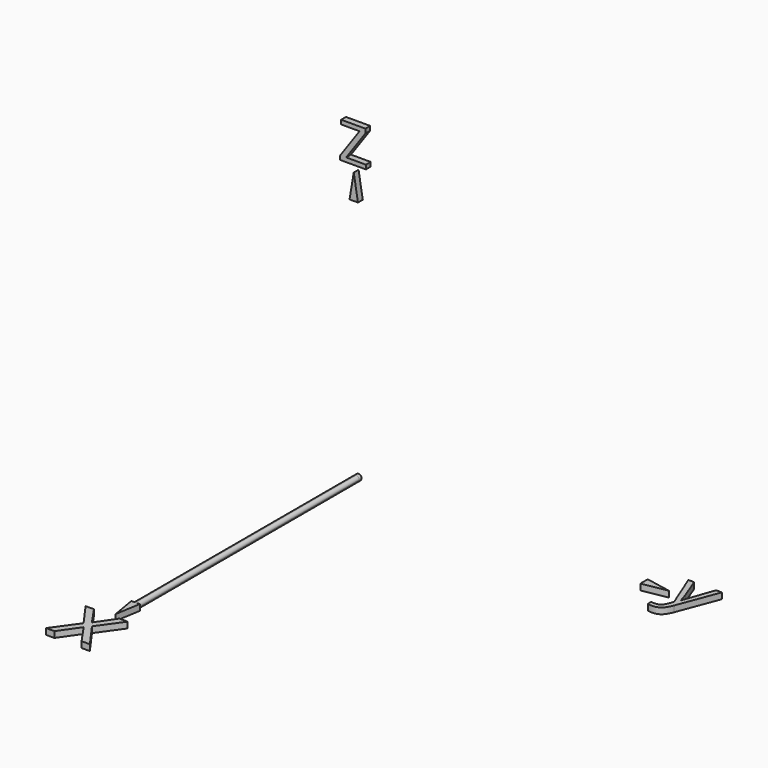
from build123d import *

# Parameters (mm, degrees)
F1_TEXT_SIZE   = 11.1111111111
F3_DEPTH       = 0.5
F0_TEXT_SIZE   = 15.0063579108
F4_DEPTH       = 1
F0_TEXT_SIZE_2 = 11.1111111111
F5_DEPTH       = 1
F6_DEPTH       = 47
F10_DEPTH      = 0.5
F11_DEPTH      = 0.5


# Not quite as in the source:
# - the program builds the solid bodies; features that only make, move or delete a surface that nothing else refers to are left out
# - Text() gives the source's letters only with a copy of the font that has no kerning and outlines rounded to 1/6400 em; it was checked with that copy


with BuildPart() as f3:
    # F1 (on Front) → F3 (new body, symmetric)
    with BuildSketch(Plane.XZ):
        Polygon((-0.699351976, 40.8282129952), (0, 40.8282129952), (0, 45), align=None)
        Polygon((0, 45), (0, 40.8282129952), (0.699351976, 40.8282129952), align=None)
        with BuildLine():
            ThreePointArc((0.5, 0), (0.3535533906, 0.3535533906), (0, 0.5))
            ThreePointArc((0, 0.5), (-0.3535533906, -0.3535533906), (0.5, 0))
        make_face()
        with Locations((-2.7395833333, 46.0987785351)):
            Text('z', F1_TEXT_SIZE, font='Open Sans', text_align=(TextAlign.LEFT, TextAlign.BOTTOM))
    extrude(amount=F3_DEPTH, both=True)


with BuildPart() as f4:
    # F0 (on Top) → F4 (new body)
    with BuildSketch(Plane.XY):
        with Locations((-4.2674330309, -59.449518038)):
            Text('x', F0_TEXT_SIZE, font='Open Sans', text_align=(TextAlign.LEFT, TextAlign.BOTTOM))
    extrude(amount=F4_DEPTH)


with BuildPart() as f5:
    # F0 (on Top) → F5 (new body)
    with BuildSketch(Plane.XY):
        with Locations((52.6564974968, -2.7562453453)):
            Text('y', F0_TEXT_SIZE_2, font='Open Sans', text_align=(TextAlign.LEFT, TextAlign.BOTTOM))
    extrude(amount=F5_DEPTH)


with BuildPart() as f6:
    # F1 (on Front) → F6 (new body)
    with BuildSketch(Plane.XZ):
        with BuildLine():
            ThreePointArc((0.5, 0), (0.3535533906, 0.3535533906), (0, 0.5))
            ThreePointArc((0, 0.5), (-0.3535533906, -0.3535533906), (0.5, 0))
        make_face()
    extrude(amount=F6_DEPTH)

    # F0 (on Top) → F10 (join, symmetric)
    with BuildSketch(Plane.XY):
        Polygon((0, -50), (0, -45.8278653363), (-0.6972749445, -45.8278653363), align=None)
        Polygon((0.6972749445, -45.8278653363), (0, -45.8278653363), (0, -50), align=None)
    extrude(amount=F10_DEPTH, both=True)


with BuildPart() as f11:
    # F0 (on Top) → F11 (new body, symmetric)
    with BuildSketch(Plane.XY):
        Polygon((47.836772, 0.8005209702), (47.8325160452, 0), (52, 0), align=None)
        Polygon((52, 0), (47.8325160452, 0), (47.8284956715, -0.7562095214), align=None)
    extrude(amount=F11_DEPTH, both=True)


solid = Compound([f3.part, f4.part, f5.part, f6.part, f11.part])
